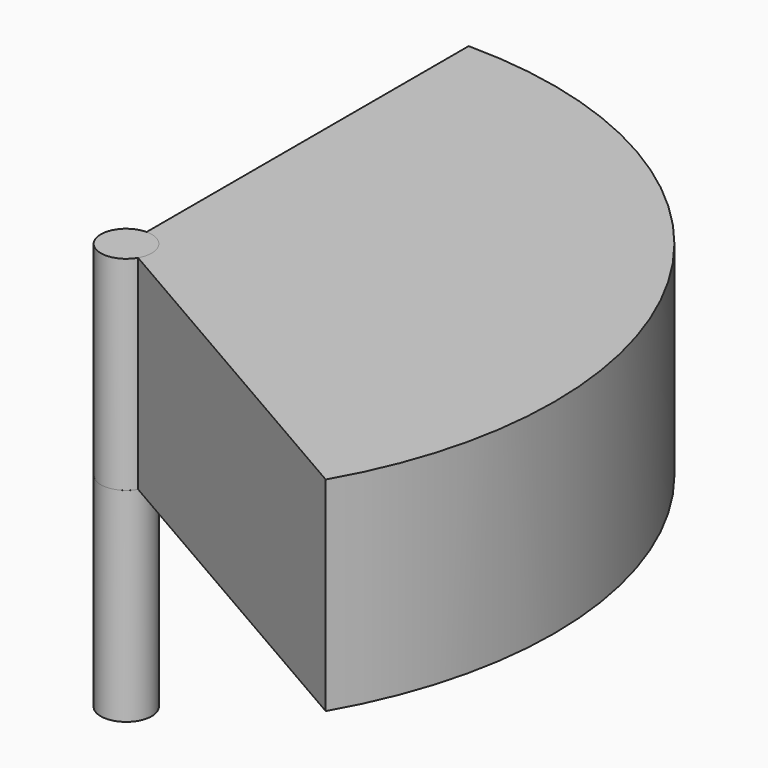
from build123d import *

# Parameters (mm, degrees)
F1_DEPTH = 50.8
F2_R     = 6.35
F3_DEPTH = 50.8
F4_DEPTH = 50.8


with BuildPart() as f1:
    # F0 (on Top) → F1 (new body)
    with BuildSketch(Plane.XY):
        with BuildLine():
            Line((0, 106.68), (0, 0))
            Line((0, 0), (92.3875900757, -53.34))
            ThreePointArc((92.3875900757, -53.34), (92.3875900757, 53.34), (0, 106.68))
        make_face()
    extrude(amount=F1_DEPTH)

    # F2 (on Top) → F4 (join)
    with BuildSketch(Plane.XY):
        Circle(F2_R)
    extrude(amount=-F4_DEPTH)


with BuildPart() as f3:
    # F2 (on Top) → F3 (new body)
    with BuildSketch(Plane.XY):
        Circle(F2_R)
    extrude(amount=F3_DEPTH)


solid = Compound([f1.part, f3.part])
